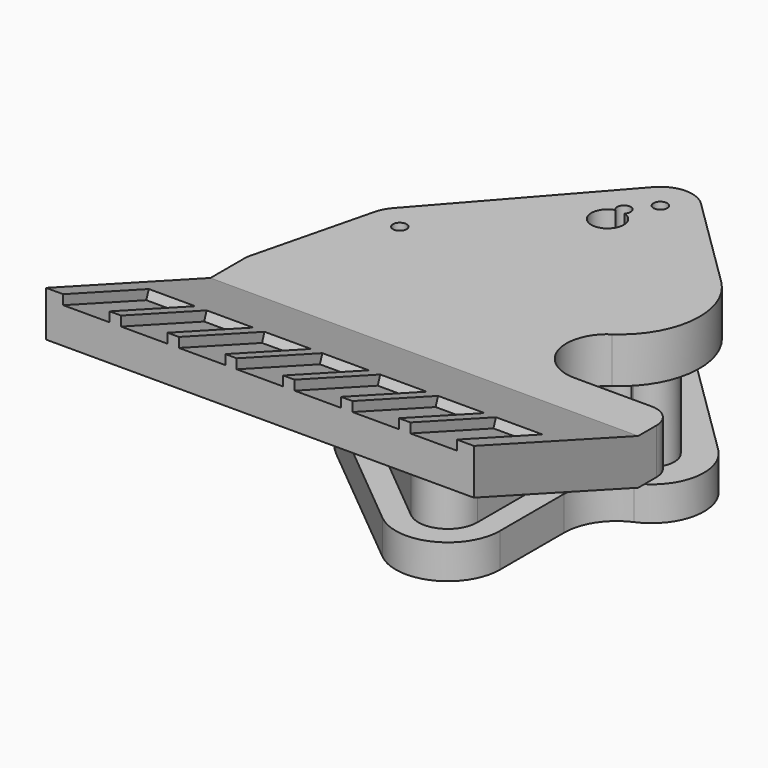
from build123d import *

# Parameters (mm, degrees)
F3_R      = 0.15
F4_DEPTH  = 4
F3_R_2    = 0.85
F6_DEPTH  = 1
F8_DEPTH  = 2.25
F10_DEPTH = 0.75
F14_W     = 1.02
F14_H     = 2.5
F15_DEPTH = 0.2


with BuildPart() as f4:
    # F3 (on Top) → F4 (new body)
    with BuildSketch(Plane.XY):
        with Locations((-3.35, -1)):
            Circle(F3_R)
    extrude(amount=F4_DEPTH)


with BuildPart() as f4b:
    # F3 (on Top) → F4, piece 2 (new body)
    with BuildSketch(Plane.XY):
        with BuildLine():
            ThreePointArc((-0.6479896557, 1.7900277778), (-0.6125199075, 1.8400064655), (-0.6, 1.9))
            ThreePointArc((-0.6, 1.9), (-0.8099935345, 2.0374800925), (-0.8520103443, 1.7900277778))
            ThreePointArc((-0.8520103443, 1.7900277778), (-0.75, 1.805), (-0.6479896557, 1.7900277778))
        make_face()
        with BuildLine():
            ThreePointArc((-0.6479896557, 1.7900277778), (-0.75, 1.805), (-0.8520103443, 1.7900277778))
            ThreePointArc((-0.8520103443, 1.7900277778), (-0.75, 1.75), (-0.6479896557, 1.7900277778))
        make_face()
        with BuildLine():
            ThreePointArc((-0.6479896557, 1.7900277778), (-0.75, 1.75), (-0.8520103443, 1.7900277778))
            ThreePointArc((-0.8520103443, 1.7900277778), (-0.9619095654, 1.1651854356), (-0.395, 1.45))
            ThreePointArc((-0.395, 1.45), (-0.4651854356, 1.6619095654), (-0.6479896557, 1.7900277778))
        make_face()
    extrude(amount=F4_DEPTH)


with BuildPart() as f4c:
    # F3 (on Top) → F4, piece 3 (new body)
    with BuildSketch(Plane.XY):
        with Locations((-0.35, 2.4)):
            Circle(F3_R)
    extrude(amount=F4_DEPTH)


with BuildPart() as f4d:
    # F3 (on Top) → F4, piece 4 (new body)
    with BuildSketch(Plane.XY):
        with Locations((2.5, -2.6)):
            Circle(F3_R_2)
    extrude(amount=F4_DEPTH)


with BuildPart() as f6:
    # F5 (on face) → F6 (new body)
    with BuildSketch(Plane.XY.offset(4)):
        with BuildLine():
            ThreePointArc((1.9858394431, -1.8458978499), (2.7430307581, -0.5560249217), (2.2269639391, 0.8478218992))
            Line((2.2269639391, 0.8478218992), (0.1407855756, 2.8991287597))
            ThreePointArc((0.1407855756, 2.8991287597), (-0.3747911939, 3.0995608599), (-0.8748864988, 2.863135146))
            Line((-0.8748864988, 2.863135146), (-3.8748864988, -0.536864854))
            ThreePointArc((-3.8748864988, -0.536864854), (-3.9698749845, -0.674800056), (-4.0293801406, -0.831350587))
            Line((-4.0293801406, -0.831350587), (-4.695, -3.5127053911))
            Line((-4.695, -3.5127053911), (-4.695, -4.5127053911))
            Line((-4.695, -4.5127053911), (4.695, -4.5127053911))
            Line((4.695, -4.5127053911), (4.695, -4.0127053911))
            ThreePointArc((4.695, -4.0127053911), (4.5485533906, -3.6591520005), (4.195, -3.5127053911))
            Line((4.195, -3.5127053911), (2.5, -3.5127053911))
            ThreePointArc((2.5, -3.5127053911), (1.6278462782, -2.869033486), (1.9858394431, -1.8458978499))
        make_face()
    extrude(amount=-F6_DEPTH)

    # F7 (on face) → F8 (join)
    with BuildSketch(Plane(origin=(0, 0, 3), x_dir=(1, 0, 0), z_dir=(0, 0, -1))):
        with BuildLine():
            ThreePointArc((0.645, 3.8677053911), (0.2746634171, 4.4513020046), (-0.411077542, 4.3647368333))
            Line((-0.411077542, 4.3647368333), (-3.429889044, 1.8679820876))
            ThreePointArc((-3.429889044, 1.8679820876), (-3.6098399318, 1.5198675017), (-3.4835090032, 1.1489138881))
            Line((-3.4835090032, 1.1489138881), (-0.75, -1.9))
            Line((-0.75, -1.9), (-0.35, -2.4))
            Line((-0.35, -2.4), (1.7282178972, -0.3565205426))
            ThreePointArc((1.7282178972, -0.3565205426), (1.840398747, 0.1893934116), (1.3776567718, 0.5))
            Line((1.3776567718, 0.5), (1.3406244266, 0.5))
            ThreePointArc((1.3406244266, 0.5), (1.0505140008, 0.0486122715), (0.645, 0.4))
            Line((0.645, 0.4), (0.645, 3.8677053911))
        make_face()
    extrude(amount=F8_DEPTH)

    # F9 (on face) → F10 (join)
    with BuildSketch(Plane(origin=(0, 0, 0.75), x_dir=(1, 0, 0), z_dir=(0, 0, -1))):
        with BuildLine():
            ThreePointArc((-3.7485538053, 2.2532777792), (-4.1598651003, 1.4614479318), (-3.8772413796, 0.6151056127))
            Line((-3.8772413796, 0.6151056127), (-0.837394606, -2.8300540641))
            ThreePointArc((-0.837394606, -2.8300540641), (-0.3730203944, -3.049592227), (0.1057294631, -2.8634767054))
            Line((0.1057294631, -2.8634767054), (2.1839473603, -0.8199972481))
            ThreePointArc((2.1839473603, -0.8199972481), (2.5083795632, 0.2096806356), (1.8363283859, 1.054571169))
            ThreePointArc((1.8363283859, 1.054571169), (1.3332379826, 1.4786553659), (1.145, 2.1091423379))
            Line((1.145, 2.1091423379), (1.145, 3.8677053911))
            ThreePointArc((1.145, 3.8677053911), (0.4875807948, 4.9037024802), (-0.7297423032, 4.7500325249))
            Line((-0.7297423032, 4.7500325249), (-3.7485538053, 2.2532777792))
        make_face()
    extrude(amount=F10_DEPTH)

    # F11: cut F4, F4b, F4c, F4d
    add(f4.part, mode=Mode.SUBTRACT)
    add(f4b.part, mode=Mode.SUBTRACT)
    add(f4c.part, mode=Mode.SUBTRACT)
    add(f4d.part, mode=Mode.SUBTRACT)

    # F13: sweep along a path in F12
    with BuildLine(Plane.YZ) as f13_path:
        Line((-9.0232299709, 5.641696688), (-4.5127053911, 4))
    # F6_face1 (on face) → F13 (sweep)
    with BuildSketch(Plane(origin=(0, -4.5127053911, 3.5), x_dir=(1, 0, 0), z_dir=(0, -1, 0))):
        Polygon((-4.695, 0.5), (-4.695, -0.5), (0, -0.5), (4.695, -0.5), (4.695, 0.5), align=None)
    sweep(path=f13_path.line)

    # F14 (on face) → F15 (cut)
    with BuildSketch(Plane(origin=(0, 0.757688968, 2.0817333304), x_dir=(1, 0, 0), z_dir=(0, 0.3420201433, 0.9396926208))):
        with Locations((-3.81, -9.1586365291)):
            Rectangle(F14_W, F14_H)
        with Locations((-2.54, -9.1586365291)):
            Rectangle(F14_W, F14_H)
        with Locations((-1.27, -9.1586365291)):
            Rectangle(F14_W, F14_H)
        with Locations((0, -9.1586365291)):
            Rectangle(F14_W, F14_H)
        with Locations((1.27, -9.1586365291)):
            Rectangle(F14_W, F14_H)
        with Locations((2.54, -9.1586365291)):
            Rectangle(F14_W, F14_H)
        with Locations((3.81, -9.1586365291)):
            Rectangle(F14_W, F14_H)
    extrude(amount=-F15_DEPTH, mode=Mode.SUBTRACT)


solid = f6.part
